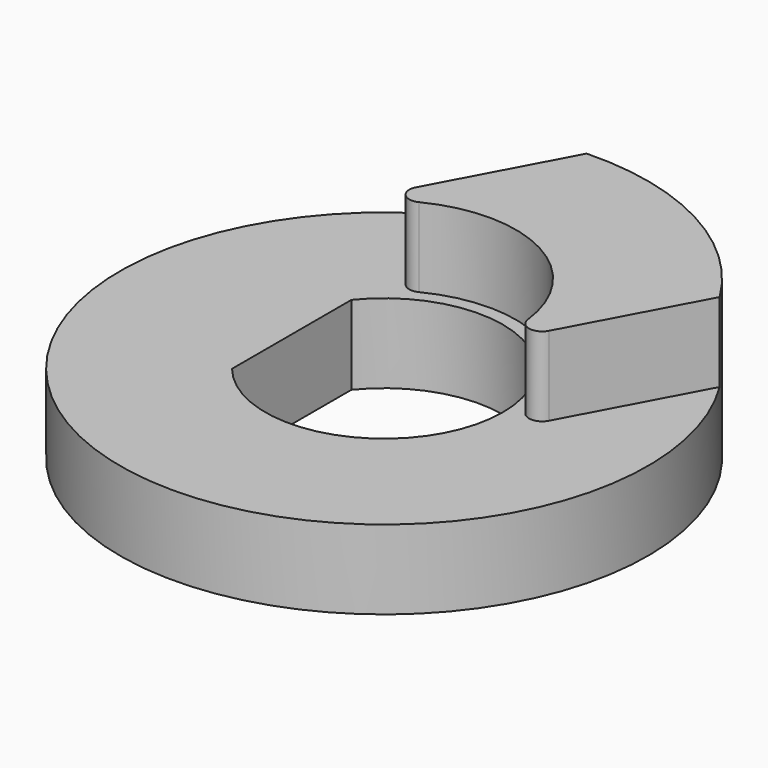
from build123d import *

# Parameters (mm, degrees)
F1_DEPTH = 3
F2_DEPTH = 6
F3_R     = 0.49999


# Not quite as in the source:
# - a fillet or chamfer is up to 0.001 mm smaller than in the source, because OpenCascade refuses the exact size


with BuildPart() as f1:
    # F0 (on Top) → F1 (new body)
    with BuildSketch(Plane.XY):
        with BuildLine():
            ThreePointArc((-0.3210767755, 9.9948441561), (-6.9566239026, -7.1836887375), (10, 0))
            ThreePointArc((10, 0), (9.616457393, 2.7429449883), (8.4952505583, 5.2754827222))
            Line((8.4952505583, 5.2754827222), (4.4081636669, -2.359680717))
            ThreePointArc((4.4081636669, -2.359680717), (2.359680717, 4.4081636669), (-4.4081636669, 2.359680717))
            Line((-4.4081636669, 2.359680717), (-0.3210767755, 9.9948441561))
        make_face()
        with BuildLine():
            ThreePointArc((-3.5, 2.8284271247), (4.5, 0), (-3.5, -2.8284271247))
            Line((-3.5, -2.8284271247), (-3.5, 2.8284271247))
        make_face(mode=Mode.SUBTRACT)
        with BuildLine():
            Line((4.4081636669, -2.359680717), (8.4952505583, 5.2754827222))
            ThreePointArc((8.4952505583, 5.2754827222), (4.7193614339, 8.8163273338), (-0.3210767755, 9.9948441561))
            Line((-0.3210767755, 9.9948441561), (-4.4081636669, 2.359680717))
            ThreePointArc((-4.4081636669, 2.359680717), (2.359680717, 4.4081636669), (4.4081636669, -2.359680717))
        make_face()
    extrude(amount=F1_DEPTH)

    # F0 (on Top) → F2 (join)
    with BuildSketch(Plane.XY):
        with BuildLine():
            Line((4.4081636669, -2.359680717), (8.4952505583, 5.2754827222))
            ThreePointArc((8.4952505583, 5.2754827222), (4.7193614339, 8.8163273338), (-0.3210767755, 9.9948441561))
            Line((-0.3210767755, 9.9948441561), (-4.4081636669, 2.359680717))
            ThreePointArc((-4.4081636669, 2.359680717), (2.359680717, 4.4081636669), (4.4081636669, -2.359680717))
        make_face()
    extrude(amount=F2_DEPTH)

    # F3 (radius 0.5 in the source; OpenCascade refuses exactly that, so slightly less here)
    f3_edges = [f1.edges().sort_by_distance(p)[0] for p in [
        (-4.408164, 2.359681, 4.5),
        (4.408164, -2.359681, 4.5),
    ]]
    fillet(f3_edges, radius=F3_R)


solid = f1.part
